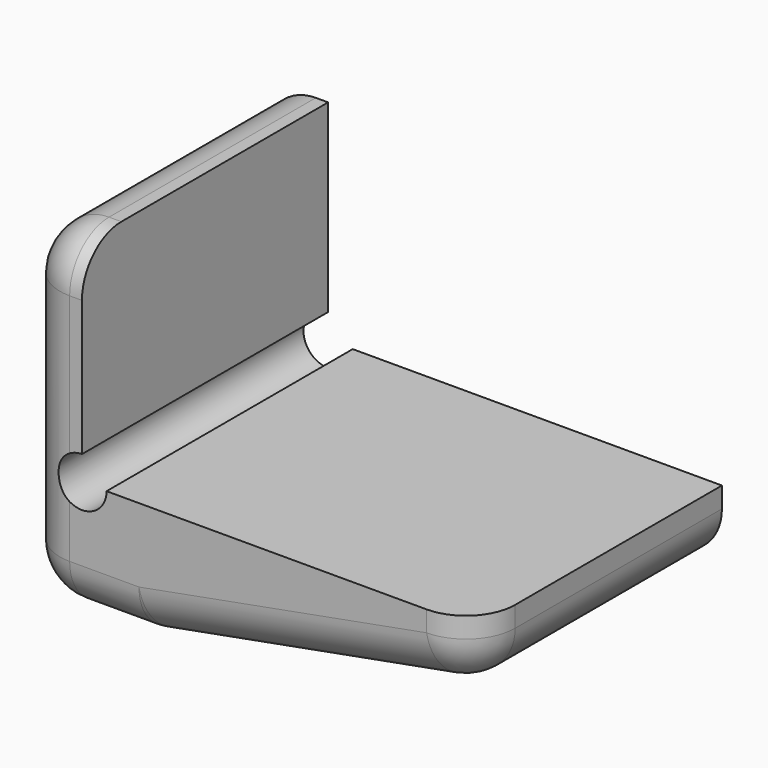
from build123d import *

# Parameters (mm, degrees)
F1_DEPTH     = 25
F2_T1_DEPTH  = 19
F2_T3_DEPTH  = 23.7645438744
F2_T5_DEPTH  = 11.6727317873
F2_T7_DEPTH  = 11
F2_T9_DEPTH  = 5.6327516516
F2_T12_ANGLE = 79.5085229877
F2_T14_ANGLE = 90
F2_T16_ANGLE = 90
F2_T18_ANGLE = 10.4914770123


# Not quite as in the source:
# - a fillet or chamfer that OpenCascade refuses, or shapes differently, is made with other operations: its cross-section is extruded or revolved along the edge and cut away or added


with BuildPart() as f1:
    # F0 (on Front) → F1 (new body)
    with BuildSketch(Plane.XZ):
        with BuildLine():
            Line((32, 0), (2, 0))
            ThreePointArc((2, 0), (-1.4142135624, -1.4142135624), (0, 2))
            Line((0, 2), (0, 17))
            Line((0, 17), (-1, 17))
            ThreePointArc((-1, 17), (-3.8284271247, 15.8284271247), (-5, 13))
            Line((-5, 13), (-5, -6))
            ThreePointArc((-5, -6), (-3.8284271247, -8.8284271247), (-1, -10))
            Line((-1, -10), (4.6327516516, -10))
            ThreePointArc((4.6327516516, -10), (4.9984618649, -9.9832469218), (5.3611086923, -9.9331280199))
            Line((5.3611086923, -9.9331280199), (28.7283570407, -5.6058598073))
            ThreePointArc((28.7283570407, -5.6058598073), (31.0751770813, -4.2307165251), (32, -1.6727317873))
            Line((32, -1.6727317873), (32, 0))
        make_face()
    extrude(amount=F1_DEPTH)

    # F2: fillet of radius 4 on 9 edges, made by hand

    # F2_s2 → F2_t1 (cut)
    with BuildSketch(Plane.XY.offset(-6)):
        with BuildLine():
            ThreePointArc((-5, -21), (-3.8284271247, -23.8284271247), (-1, -25))
            Line((-1, -25), (-5, -25))
            Line((-5, -25), (-5, -21))
        make_face()
    extrude(amount=F2_T1_DEPTH, mode=Mode.SUBTRACT)

    # F2_s4 → F2_t3 (cut)
    with BuildSketch(Plane(origin=(3.4048752706, 0, 0.6305324575), x_dir=(0, 1, 0), z_dir=(0.983282005, 0, 0.1820892602))):
        with BuildLine():
            ThreePointArc((-21, -10.7432663508), (-23.8284271247, -9.5716934755), (-25, -6.7432663508))
            Line((-25, -6.7432663508), (-25, -10.7432663508))
            Line((-25, -10.7432663508), (-21, -10.7432663508))
        make_face()
    extrude(amount=F2_T3_DEPTH, mode=Mode.SUBTRACT)

    # F2_s6 → F2_t5 (cut)
    with BuildSketch(Plane.XY.offset(-1.6727317873)):
        with BuildLine():
            ThreePointArc((32, -21), (30.8284271247, -23.8284271247), (28, -25))
            Line((28, -25), (32, -25))
            Line((32, -25), (32, -21))
        make_face()
    extrude(amount=F2_T5_DEPTH, mode=Mode.SUBTRACT)

    # F2_s8 → F2_t7 (cut)
    with BuildSketch(Plane.YZ.offset(-1)):
        with BuildLine():
            ThreePointArc((-21, 17), (-23.8284271247, 15.8284271247), (-25, 13))
            Line((-25, 13), (-25, 17))
            Line((-25, 17), (-21, 17))
        make_face()
    extrude(amount=F2_T7_DEPTH, mode=Mode.SUBTRACT)

    # F2_s10 → F2_t9 (cut)
    with BuildSketch(Plane.YZ.offset(-1)):
        with BuildLine():
            ThreePointArc((-21, -10), (-23.8284271247, -8.8284271247), (-25, -6))
            Line((-25, -6), (-25, -10))
            Line((-25, -10), (-21, -10))
        make_face()
    extrude(amount=F2_T9_DEPTH, mode=Mode.SUBTRACT)

    # F2_s11 → F2_t12 (revolve, cut)
    with BuildSketch(Plane(origin=(26.772123619, 0, 4.9578006702), x_dir=(0, 1, 0), z_dir=(-0.983282005, 0, -0.1820892602))):
        with BuildLine():
            ThreePointArc((-21, 10.7432663508), (-23.8284271247, 9.5716934755), (-25, 6.7432663508))
            Line((-25, 6.7432663508), (-25, 10.7432663508))
            Line((-25, 10.7432663508), (-21, 10.7432663508))
        make_face()
    revolve(axis=Axis((28, -25, -1.6727317873), (0, -1, 0)), revolution_arc=F2_T12_ANGLE, mode=Mode.SUBTRACT)

    # F2_s13 → F2_t14 (revolve, cut)
    with BuildSketch(Plane.YZ.offset(-1)):
        with BuildLine():
            ThreePointArc((-21, 17), (-23.8284271247, 15.8284271247), (-25, 13))
            Line((-25, 13), (-25, 17))
            Line((-25, 17), (-21, 17))
        make_face()
    revolve(axis=Axis((-1, -25, 13), (0, -1, 0)), revolution_arc=F2_T14_ANGLE, mode=Mode.SUBTRACT)

    # F2_s15 → F2_t16 (revolve, cut)
    with BuildSketch(Plane.XY.offset(-6)):
        with BuildLine():
            ThreePointArc((-5, -21), (-3.8284271247, -23.8284271247), (-1, -25))
            Line((-1, -25), (-5, -25))
            Line((-5, -25), (-5, -21))
        make_face()
    revolve(axis=Axis((-1, -25, -6), (0, -1, 0)), revolution_arc=F2_T16_ANGLE, mode=Mode.SUBTRACT)

    # F2_s17 → F2_t18 (revolve, cut)
    with BuildSketch(Plane.YZ.offset(4.6327516516)):
        with BuildLine():
            ThreePointArc((-21, -10), (-23.8284271247, -8.8284271247), (-25, -6))
            Line((-25, -6), (-25, -10))
            Line((-25, -10), (-21, -10))
        make_face()
    revolve(axis=Axis((4.6327516516, -25, -6), (0, -1, 0)), revolution_arc=F2_T18_ANGLE, mode=Mode.SUBTRACT)


solid = f1.part
